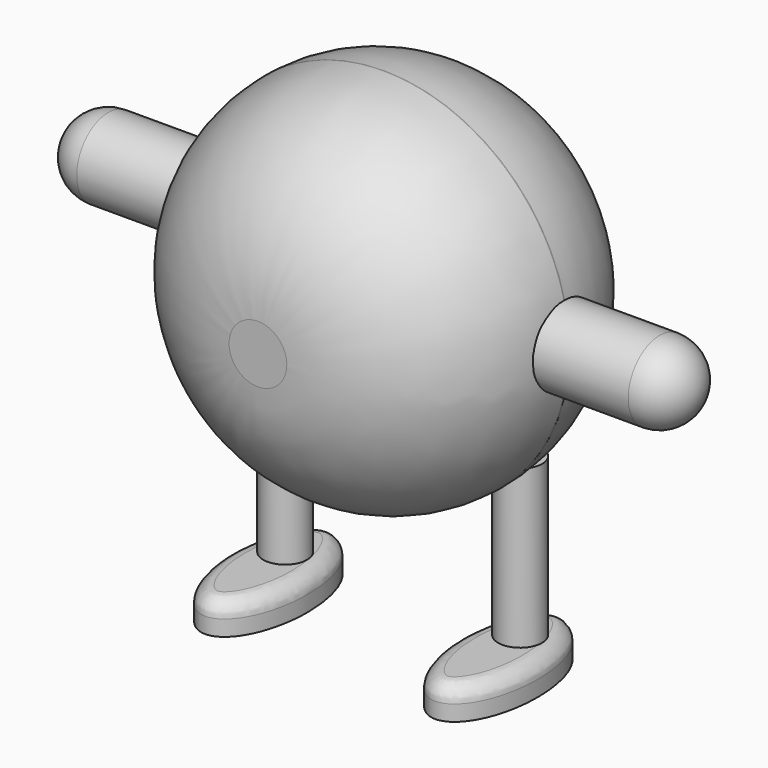
from build123d import *

# Parameters (mm, degrees)
F1_DEPTH      = 5.08
F2_R          = 2.54
F2_2_R        = 2.54
F3_R          = 3.5284597722
F4_DEPTH      = 25.4
F3_R_2        = 3.5284608279
F5_R          = 29.9123842009
F6_DEPTH      = 25.4
F7_DEPTH      = 25.4
F8_S5_R       = 3.5284597722
F8_T6_DEPTH   = 337695
F8_2_T2_ANGLE = 352.1873774243
F8_2_T4_ANGLE = 249.5405171679
F9_R          = 6.35
F10_DEPTH     = 50.8
F11_R         = 6.35
F12_R         = 6.35
F13_DEPTH     = 50.8
F14_R         = 6.35


# Not quite as in the source:
# - a fillet or chamfer that OpenCascade refuses, or shapes differently, is made with other operations: its cross-section is extruded or revolved along the edge and cut away or added


with BuildPart() as f1:
    # F0 (on Top) → F1 (new body)
    with BuildSketch(Plane.XY):
        with BuildLine():
            add(Edge.make_bspline(
                [(-18.6551132891, -12.7), (-12.3051132891, -12.7), (-12.3051132891, 0)],
                knots=[0, 0, 0, 1.5707963268, 1.5707963268, 1.5707963268], degree=2, weights=[1, 0.7071067812, 1]))
            add(Edge.make_bspline(
                [(-12.3051132891, 0), (-12.3051132891, 30.6605122421), (-23.1452413496, 8.9802561211), (-33.9853694101, -12.7), (-18.6551132891, -12.7)],
                knots=[1.5707963268, 1.5707963268, 1.5707963268, 3.926990817, 3.926990817, 6.2831853072, 6.2831853072, 6.2831853072], degree=2, weights=[1, 0.3826834324, 1, 0.3826834324, 1]))
        make_face()
    extrude(amount=F1_DEPTH)

    # F2
    f2_edges = [f1.edges().sort_by_distance(p)[0] for p in [
        (-23.761235, 7.549841, 5.08),
        (-14.164985, -8.980256, 5.08),
    ]]
    fillet(f2_edges, radius=F2_R)


with BuildPart() as f1b:
    # F0 (on Top) → F1, piece 2 (new body)
    with BuildSketch(Plane.XY):
        with BuildLine():
            add(Edge.make_bspline(
                [(18.4274641449, -12.7), (33.757720266, -12.7), (22.9175922054, 8.9802561211), (12.0774641449, 30.6605122421), (12.0774641449, 0)],
                knots=[0, 0, 0, 2.3561944902, 2.3561944902, 4.7123889804, 4.7123889804, 4.7123889804], degree=2, weights=[1, 0.3826834324, 1, 0.3826834324, 1]))
            add(Edge.make_bspline(
                [(12.0774641449, 0), (12.0774641449, -12.7), (18.4274641449, -12.7)],
                knots=[4.7123889804, 4.7123889804, 4.7123889804, 6.2831853072, 6.2831853072, 6.2831853072], degree=2, weights=[1, 0.7071067812, 1]))
        make_face()
    extrude(amount=F1_DEPTH)

    # F2#2
    f2_2_edges = [f1b.edges().sort_by_distance(p)[0] for p in [
        (23.533586, 7.549841, 5.08),
        (13.937336, -8.980256, 5.08),
    ]]
    fillet(f2_2_edges, radius=F2_2_R)


with BuildPart() as f4:
    # F3 (on face) → F4 (new body)
    with BuildSketch(Plane.XY.offset(5.08)):
        with Locations((-18.7353696674, 3.5060022492)):
            Circle(F3_R)
    extrude(amount=F4_DEPTH)

    # F5 (on Front) → F6 (join)
    with BuildSketch(Plane.XZ):
        with Locations((0, 50.9765781462)):
            Circle(F5_R)
    extrude(amount=F6_DEPTH)


with BuildPart() as f4b:
    # F3 (on face) → F4, piece 2 (new body)
    with BuildSketch(Plane.XY.offset(5.08)):
        with Locations((18.5067411512, 4.2928075418)):
            Circle(F3_R_2)
    extrude(amount=F4_DEPTH)


with BuildPart() as f7:
    # F7 (new): a face of the model
    f7_faces = [f4.part.faces().sort_by_distance(p)[0] for p in [
        (0.0149396999, 0, 50.9940652934),
    ]]
    extrude(f7_faces, amount=F7_DEPTH)

    # F8#2: fillet of radius 25.4 on 2 edges, made by hand

    # F8_2_s1 → F8_2_t2 (revolve, cut)
    with BuildSketch(Plane.XY.offset(50.9765781462)):
        with BuildLine():
            ThreePointArc((29.9123842009, 0), (22.472896443, 17.9605122421), (4.5123842009, 25.4))
            Line((4.5123842009, 25.4), (29.9123842009, 25.4))
            Line((29.9123842009, 25.4), (29.9123842009, 0))
        make_face()
    revolve(axis=Axis((0, 25.4, 50.9765781462), (0, -1, 0)), revolution_arc=F8_2_T2_ANGLE, mode=Mode.SUBTRACT)

    # F8_2_s3 → F8_2_t4 (revolve, cut)
    with BuildSketch(Plane(origin=(16.6945993208, 0, 6.228402433), x_dir=(0, 1, 0), z_dir=(0.936919607, 0, 0.3495449185))):
        with BuildLine():
            ThreePointArc((0, 77.6733397624), (17.9605122421, 70.2338520045), (25.4, 52.2733397624))
            Line((25.4, 52.2733397624), (25.4, 77.6733397624))
            Line((25.4, 77.6733397624), (0, 77.6733397624))
        make_face()
    revolve(axis=Axis((0, 25.4, 50.9765781462), (0, -1, 0)), revolution_arc=F8_2_T4_ANGLE, mode=Mode.SUBTRACT)


with BuildPart() as f4_1:
    add(f4.part)

    # F8: fillet of radius 25.4 on 1 edges, made by hand


with BuildPart() as f8_tool2:
    # F8_s3 → F8_t4 (revolve)
    with BuildSketch(Plane.XY.offset(50.9765781462)):
        with BuildLine():
            ThreePointArc((29.9127842009, 0.0009656854), (22.472896443, -17.9605122421), (4.5114185154, -25.4004))
            Line((4.5114185154, -25.4004), (4.5114185154, -27.9405365685))
            ThreePointArc((4.5114185154, -27.9405365685), (17.2119013581, -27.9401365685), (29.9123842009, -27.9401365685))
            Line((29.9123842009, -27.9401365685), (32.4525207694, -25.4))
            ThreePointArc((32.4525207694, -25.4), (32.4525207694, -12.6995171573), (32.4529207694, 0.0009656854))
            Line((32.4529207694, 0.0009656854), (29.9127842009, 0.0009656854))
        make_face()
    revolve(axis=Axis((0, -25.4, 50.9765781462), (0, -1, 0)))

    # F8_s5 → F8_t6 (cut, symmetric)
    with BuildSketch(Plane.XY.offset(51)):
        with Locations((-18.7353696674, 3.5060022492)):
            Circle(F8_S5_R)
    extrude(amount=F8_T6_DEPTH, both=True, mode=Mode.SUBTRACT)


with BuildPart() as f4_2:
    add(f4_1.part)

    # F8_t1: cut F8_tool2
    add(f8_tool2.part, mode=Mode.SUBTRACT)


with BuildPart() as f10:
    # F9 (on Right) → F10 (new body)
    with BuildSketch(Plane.YZ):
        with Locations((0, 51.4177073274)):
            Circle(F9_R)
    extrude(amount=F10_DEPTH)

    # F11
    f11_edges = [f10.edges().sort_by_distance(p)[0] for p in [
        (50.8, -6.35, 51.417707),
    ]]
    fillet(f11_edges, radius=F11_R)


with BuildPart() as f13:
    # F12 (on Right) → F13 (new body)
    with BuildSketch(Plane.YZ):
        with Locations((0, 54.1263227366)):
            Circle(F12_R)
    extrude(amount=-F13_DEPTH)

    # F14
    f14_edges = [f13.edges().sort_by_distance(p)[0] for p in [
        (-50.8, -6.35, 54.126323),
    ]]
    fillet(f14_edges, radius=F14_R)


solid = Compound([f1.part, f1b.part, f4b.part, f7.part, f4_2.part, f10.part, f13.part])
